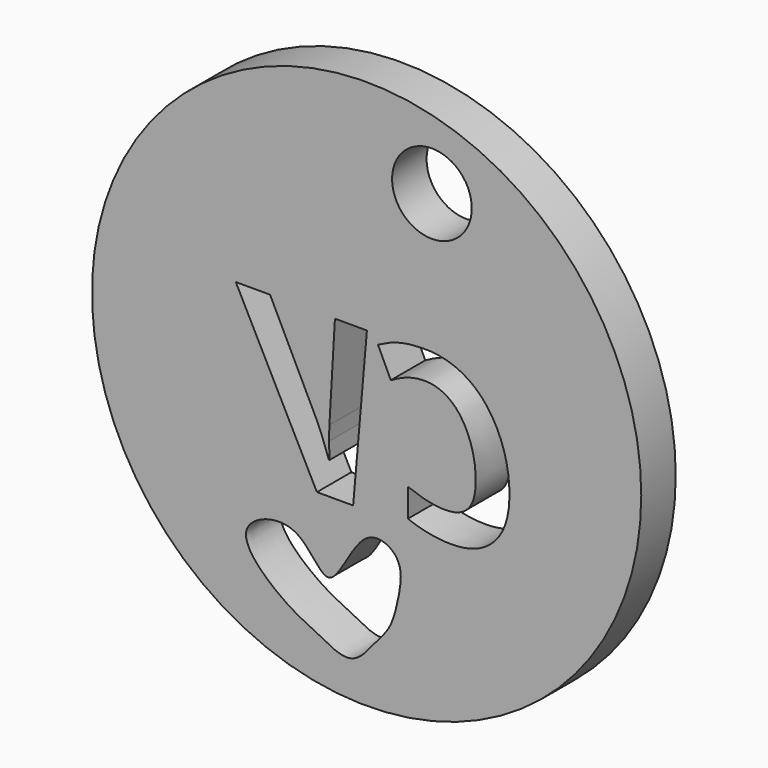
from build123d import *

# Parameters (mm, degrees)
F0_R         = 13.7
F1_DEPTH     = 2.15
F2_R         = 1.9876145449
F3_DEPTH     = 2.15
F4_TEXT_SIZE = 11.0794220948
F5_DEPTH     = 2.15
F7_DEPTH     = 2.15


# Not quite as in the source:
# - Text() gives the source's letters only with a copy of the font that has no kerning and outlines rounded to 1/6400 em; it was checked with that copy


with BuildPart() as f1:
    # F0 (on Front) → F1 (new body)
    with BuildSketch(Plane.XZ):
        with Locations((-47.333329916, 45.8073951304)):
            Circle(F0_R)
    extrude(amount=F1_DEPTH)

    # F2 (on face) → F3 (cut, through all)
    with BuildSketch(Plane(origin=(0, 0, 0), x_dir=(-1, 0, 0), z_dir=(0, 1, 0))):
        with Locations((44.0764203668, 55.6620359421)):
            Circle(F2_R)
    extrude(amount=-F3_DEPTH, mode=Mode.SUBTRACT)

    # F4 (on face) → F5 (cut, through all)
    with BuildSketch(Plane(origin=(0, 0, 0), x_dir=(-1, 0, 0), z_dir=(0, 1, 0))):
        with Locations((39.5440757275, 40.688958019)):
            Text('CV', F4_TEXT_SIZE, font='Open Sans', font_style=FontStyle.BOLDITALIC, text_align=(TextAlign.LEFT, TextAlign.BOTTOM))
    extrude(amount=-F5_DEPTH, mode=Mode.SUBTRACT)

    # F6 (on Front) → F7 (cut, through all)
    with BuildSketch(Plane.XZ):
        with BuildLine():
            add(Edge.make_bspline(
                [(-49.2053441703, 37.1306762099), (-49.6815772126, 37.0463449125), (-50.6104553822, 39.4748996785), (-54.5077016243, 38.0552230894), (-51.5521322056, 35.2811671933), (-49.7988742981, 34.5203352296), (-48.0000267923, 33.4923154402), (-46.8724473682, 35.1407191975), (-46.1189894995, 35.8476034649), (-45.7105873554, 37.4005640044), (-45.4434721257, 39.2353358), (-47.69566245, 40.2288840831), (-48.6646779268, 37.226417332), (-49.2053441703, 37.1306762099)],
                knots=[0, 0, 0, 0, 0.098833585, 0.2004322534, 0.3104973669, 0.408023764, 0.4915005916, 0.5749108083, 0.6418714122, 0.723062734, 0.8072612359, 0.8877944653, 1, 1, 1, 1], degree=3))
        make_face()
    extrude(amount=F7_DEPTH, mode=Mode.SUBTRACT)


solid = f1.part
